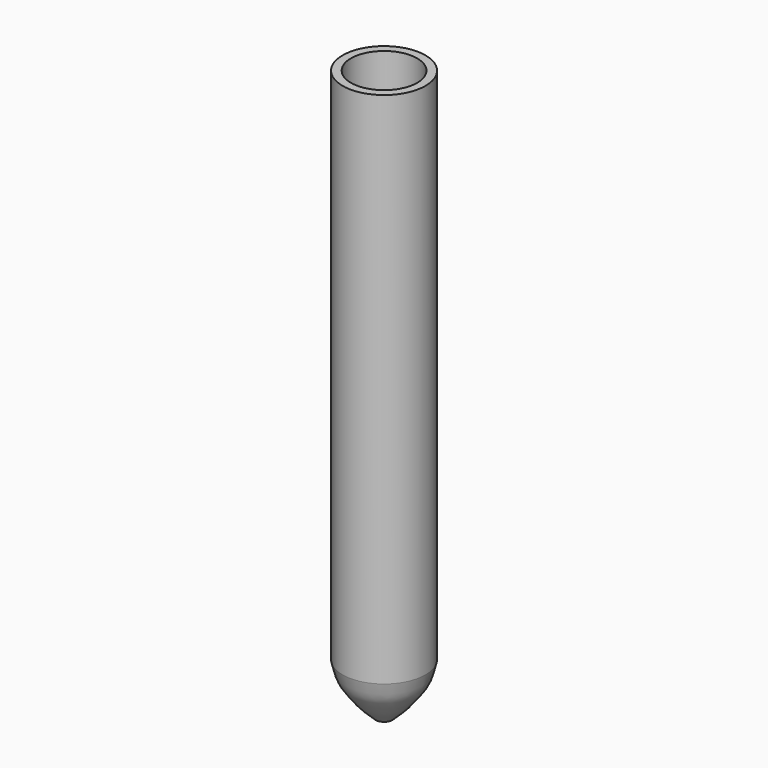
from build123d import *


# Not quite as in the source:
# - ends of sketch curves that miss each other by under 0.0002 mm in the source are joined
# - the dataset's text gives a spline's control points without its knots; the knots are read off the source's solid


with BuildPart() as f1:
    # F0 (on Front) → F1 (revolve)
    with BuildSketch(Plane.XZ):
        with BuildLine():
            Line((4.9820518226, -10.0632566027), (4.9820518226, 52.5000020862))
            Line((4.9820518226, 52.5000020862), (3.9820518226, 52.5000020862))
            Line((3.9820518226, 52.5000020862), (3.9820518226, -9.9692390828))
            add(Edge.make_bspline(
                [(3.9820518226, -9.9692390828), (3.8960358888, -10.4133868694), (3.6962547807, -11.1652142126), (3.4266604083, -11.7784613334), (3.2062152713, -12.156226186), (3.0377783729, -12.4015351386), (2.8899168759, -12.5940484972), (2.7647081274, -12.7518079956), (2.6663536541, -12.8756125644), (2.5669826855, -13.0038999912), (2.4440592341, -13.1657675618), (2.2976929411, -13.3601854659), (2.1154886116, -13.5942955714), (1.8330437933, -13.9350790006), (1.4718408507, -14.3286342999), (1.0925952968, -14.7020141969), (0.982038116, -14.8084871475)],
                knots=[0.0077245823, 0.0077245823, 0.0077245823, 0.0077245823, 0.125, 0.25, 0.3125, 0.375, 0.4375, 0.46875, 0.5, 0.53125, 0.5625, 0.625, 0.6875, 0.75, 0.875, 0.9205191269, 0.9205191269, 0.9205191269, 0.9205191269], degree=3))
            Line((0.982038116, -14.8084871475), (0.9820518317, -16.1742437631))
            add(Edge.make_bspline(
                [(4.9820518226, -10.0632566027), (4.5882822014, -12.1806906536), (3.2919426675, -13.5627068416), (2.6173668936, -14.696707597), (0.9820518317, -16.1742437631)],
                knots=[0, 0, 0, 0, 0.5054789039, 1, 1, 1, 1], degree=3))
        make_face()
    revolve(axis=Axis((-0.0179481774, 0, 18.1628791615), (0, 0, -1)))


solid = f1.part
